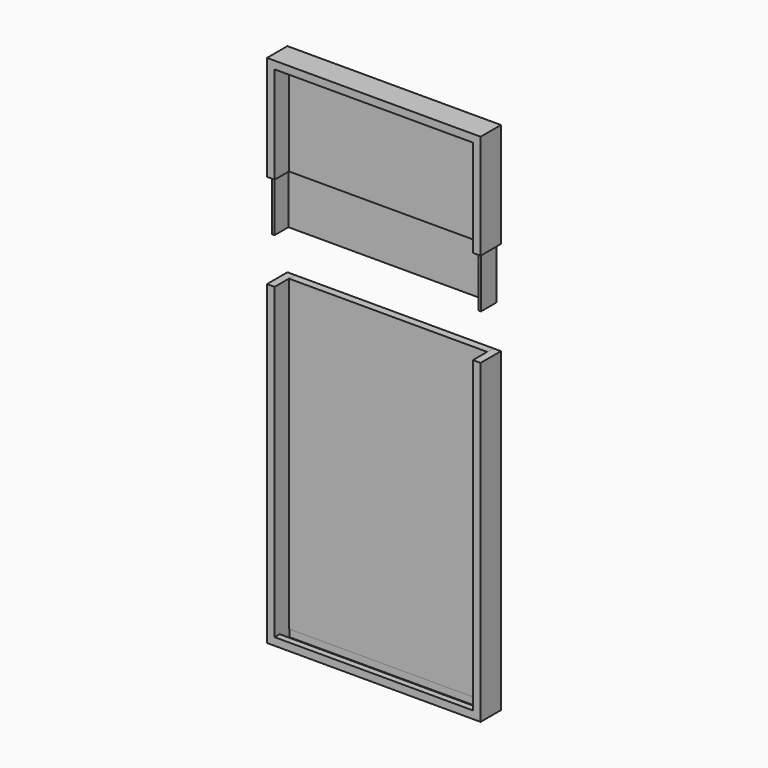
from build123d import *

# Parameters (mm, degrees)
F0_W     = 77.8
F0_H     = 121.0094395578
F1_DEPTH = 3
F0_H_2   = 38.1
F2_DEPTH = 10
F3_W     = 77.8
F3_H     = 4.8423867873
F4_DEPTH = 25
F5_W     = 77.8
F5_H     = 0.8
F6_DEPTH = 20


with BuildPart() as f1:
    # F0 (on Front) → F1 (new body)
    with BuildSketch(Plane.XZ):
        with Locations((-0.2750502467, 0.0047197789)):
            Rectangle(F0_W, F0_H)
    extrude(amount=F1_DEPTH)


with BuildPart() as f1b:
    # F0 (on Front) → F1, piece 2 (new body)
    with BuildSketch(Plane.XZ):
        with Locations((-0.2750502467, 116.5858240604)):
            Rectangle(F0_W, F0_H_2)
    extrude(amount=F1_DEPTH)


with BuildPart() as f2:
    # F0 (on Front) → F2 (new body)
    with BuildSketch(Plane.XZ):
        Polygon((38.6249497533, 60.5094395578), (38.6249497533, -60.5), (-39.1750502467, -60.5), (-39.1750502467, 60.5094395578), (-42.1750502467, 60.5094395578), (-42.1750502467, -63.5), (41.6249497533, -63.5), (41.6249497533, 60.5094395578), align=None)
    extrude(amount=F2_DEPTH)

    # F3 (on face) → F4 (cut)
    with BuildSketch(Plane(origin=(0, 0, -63.5), x_dir=(1, 0, 0), z_dir=(0, 0, -1))):
        with Locations((-0.2750502467, 5.085134937)):
            Rectangle(F3_W, F3_H)
    extrude(amount=-F4_DEPTH, mode=Mode.SUBTRACT)


with BuildPart() as f2b:
    # F0 (on Front) → F2, piece 2 (new body)
    with BuildSketch(Plane.XZ):
        Polygon((38.6249497533, 135.6358240604), (38.6249497533, 97.5358240604), (41.6249497533, 97.5358240604), (41.6249497533, 138.6358240604), (-42.1750502467, 138.6358240604), (-42.1750502467, 97.5358240604), (-39.1750502467, 97.5358240604), (-39.1750502467, 135.6358240604), align=None)
    extrude(amount=F2_DEPTH)


with BuildPart() as f6:
    # F5 (on face) → F6 (new body)
    with BuildSketch(Plane(origin=(0, 0, 97.5358240604), x_dir=(1, 0, 0), z_dir=(0, 0, -1))):
        with Locations((-0.2750502467, 1.6)):
            Rectangle(F5_W, F5_H)
        Polygon((39.8249497533, 2), (38.6249497533, 2), (38.6249497533, 1.2), (39.8249497533, 1.2), (40.8249497533, 1.2), (40.8249497533, 8.8), (39.8249497533, 8.8), align=None)
        Polygon((-39.1750502467, 2), (-40.1750502467, 2), (-40.1750502467, 8.8), (-41.1750502467, 8.8), (-41.1750502467, 1.2), (-39.1750502467, 1.2), align=None)
    extrude(amount=F6_DEPTH)


solid = Compound([f1.part, f1b.part, f2.part, f2b.part, f6.part])
